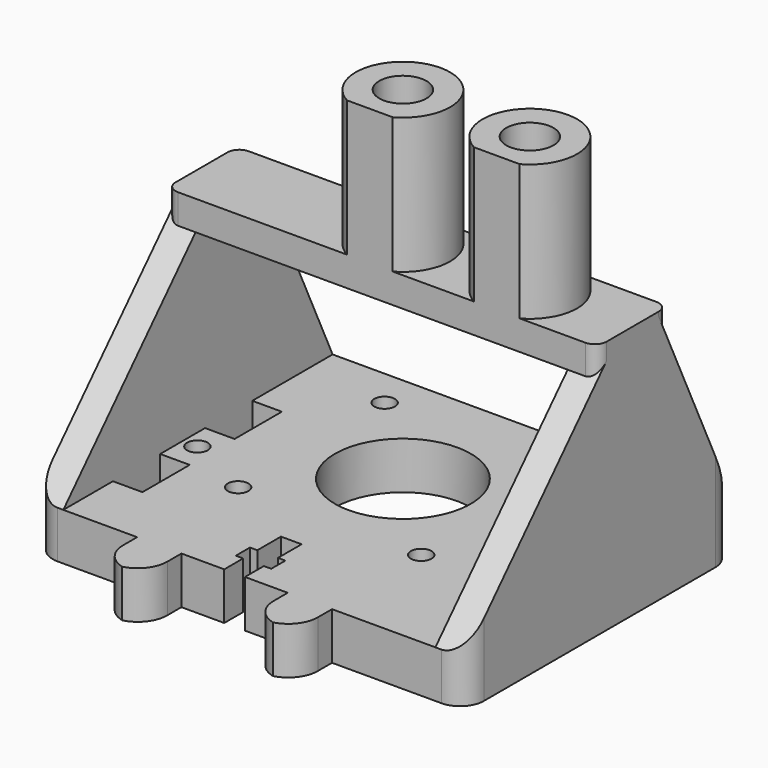
from build123d import *

# Parameters (mm, degrees)
F0_W         = 5
F0_H         = 10
F0_R         = 1.75
F0_R_2       = 4
F0_R_3       = 11.5
F0_W_2       = 7.5
F0_H_2       = 8
F1_DEPTH     = 8
F3_DEPTH     = 30
F4_W         = 5
F4_H         = 15
F4_W_2       = 63
F4_R         = 4
F5_DEPTH     = 5
F6_R         = 4
F7_DEPTH     = 23
F9_DEPTH     = 73
F10_R        = 4
F11_R        = 2
F12_T1_DEPTH = 33


# Not quite as in the source:
# - a fillet or chamfer that OpenCascade refuses, or shapes differently, is made with other operations: its cross-section is extruded or revolved along the edge and cut away or added


with BuildPart() as f1:
    # F0 (on Top) → F1 (new body)
    with BuildSketch(Plane.XY):
        Polygon((0, 57), (0, 0), (22.5, 0), (30, 0), (37.25, 0), (37.25, 4), (36, 4), (36, 7), (37.25, 7), (37.25, 12), (40.75, 12), (40.75, 7), (42, 7), (42, 4), (40.75, 4), (40.75, 0), (48, 0), (55.5, 0), (73, 0), (73, 57), align=None)
        with Locations((7.5, 15.5)):
            Rectangle(F0_W, F0_H, mode=Mode.SUBTRACT)
        with Locations((23, 19.5)):
            Circle(F0_R, mode=Mode.SUBTRACT)
        with Locations((54, 19.5)):
            Circle(F0_R, mode=Mode.SUBTRACT)
        with Locations((65.5, 15.5)):
            Rectangle(F0_W, F0_H, mode=Mode.SUBTRACT)
        with Locations((7.5, 25.25)):
            Circle(F0_R, mode=Mode.SUBTRACT)
        with Locations((7.5, 35)):
            Rectangle(F0_W, F0_H, mode=Mode.SUBTRACT)
        with Locations((17, 35)):
            Circle(F0_R_2, mode=Mode.SUBTRACT)
        with Locations((23, 50.5)):
            Circle(F0_R, mode=Mode.SUBTRACT)
        with Locations((38.5, 35)):
            Circle(F0_R_3, mode=Mode.SUBTRACT)
        with Locations((65.5, 25.25)):
            Circle(F0_R, mode=Mode.SUBTRACT)
        with Locations((65.5, 35)):
            Rectangle(F0_W, F0_H, mode=Mode.SUBTRACT)
        with Locations((54, 50.5)):
            Circle(F0_R, mode=Mode.SUBTRACT)
        with Locations((51.75, -4)):
            Rectangle(F0_W_2, F0_H_2)
        with Locations((26.25, -4)):
            Rectangle(F0_W_2, F0_H_2)
    extrude(amount=-F1_DEPTH)

    # F2 (on Top) → F3 (join)
    with BuildSketch(Plane.XY):
        Polygon((0, 57), (0, 0), (5, 0), (5, 10.5), (5, 20.5), (5, 30), (5, 40), (5, 57), align=None)
        Polygon((73, 57), (68, 57), (68, 40), (68, 30), (68, 20.5), (68, 10.5), (68, 0), (73, 0), align=None)
    extrude(amount=F3_DEPTH)

    # F4 (on face) → F5 (join)
    with BuildSketch(Plane.XY.offset(30)):
        with Locations((2.5, 35.5)):
            Rectangle(F4_W, F4_H)
        with Locations((36.5, 35.5)):
            Rectangle(F4_W_2, F4_H)
        with Locations((17, 35)):
            Circle(F4_R, mode=Mode.SUBTRACT)
        with Locations((38.5, 35)):
            Circle(F4_R, mode=Mode.SUBTRACT)
        with Locations((70.5, 35.5)):
            Rectangle(F4_W, F4_H)
    extrude(amount=F5_DEPTH)

    # F6 (on face) → F7 (join)
    with BuildSketch(Plane.XY.offset(35)):
        with BuildLine():
            ThreePointArc((25, 35), (22.6568542495, 40.6568542495), (17, 43))
            ThreePointArc((17, 43), (9.2540333076, 37), (13.1270166538, 28))
            Line((13.1270166538, 28), (20.8729833462, 28))
            ThreePointArc((20.8729833462, 28), (23.8914391374, 30.9369879873), (25, 35))
        make_face()
        with Locations((17, 35)):
            Circle(F6_R, mode=Mode.SUBTRACT)
        with BuildLine():
            ThreePointArc((46.5, 35), (44.1568542495, 40.6568542495), (38.5, 43))
            ThreePointArc((38.5, 43), (30.7540333076, 37), (34.6270166538, 28))
            Line((34.6270166538, 28), (42.3729833462, 28))
            ThreePointArc((42.3729833462, 28), (45.3914391374, 30.9369879873), (46.5, 35))
        make_face()
        with Locations((38.5, 35)):
            Circle(F6_R, mode=Mode.SUBTRACT)
    extrude(amount=F7_DEPTH)

    # F8 (on face) → F9 (cut)
    with BuildSketch(Plane(origin=(0, 0, 0), x_dir=(0, -1, 0), z_dir=(-1, 0, 0))):
        Polygon((-57, 0), (-43, 30), (-57, 30), align=None)
        Polygon((0, 30), (-28, 30), (0, 0), align=None)
    extrude(amount=-F9_DEPTH, mode=Mode.SUBTRACT)

    # F10
    f10_edges = [f1.edges().sort_by_distance(p)[0] for p in [
        (0, 57, -4),
        (73, 57, -4),
        (0, 0, -4),
        (73, 0, -4),
    ]]
    fillet(f10_edges, radius=F10_R)

    # F11
    f11_edges = [f1.edges().sort_by_distance(p)[0] for p in [
        (73, 28, 32.5),
        (0, 28, 32.5),
        (0, 43, 32.5),
        (73, 43, 32.5),
    ]]
    fillet(f11_edges, radius=F11_R)

    # F12: fillet of radius 5 on 4 edges, made by hand

    # F12_s2 → F12_t1 (cut)
    with BuildSketch(Plane.XY.offset(-20.5)):
        with BuildLine():
            ThreePointArc((25, -8), (28.5355339059, -6.5355339059), (30, -3))
            Line((30, -3), (30, -8))
            Line((30, -8), (25, -8))
        make_face()
        with BuildLine():
            ThreePointArc((22.5, -3), (23.9644660941, -6.5355339059), (27.5, -8))
            Line((27.5, -8), (22.5, -8))
            Line((22.5, -8), (22.5, -3))
        make_face()
        with BuildLine():
            ThreePointArc((55.5, -3), (54.0355339059, -6.5355339059), (50.5, -8))
            Line((50.5, -8), (55.5, -8))
            Line((55.5, -8), (55.5, -3))
        make_face()
        with BuildLine():
            ThreePointArc((53, -8), (49.4644660941, -6.5355339059), (48, -3))
            Line((48, -3), (48, -8))
            Line((48, -8), (53, -8))
        make_face()
    extrude(amount=F12_T1_DEPTH, mode=Mode.SUBTRACT)


with BuildPart() as f13_1:
    # F13: instance of F1
    add(f1.part.mirror(Plane(origin=(0, 30.6667140421, 8.8934527193), x_dir=(0, -1, 0), z_dir=(-1, 0, 0))))


solid = f13_1.part
